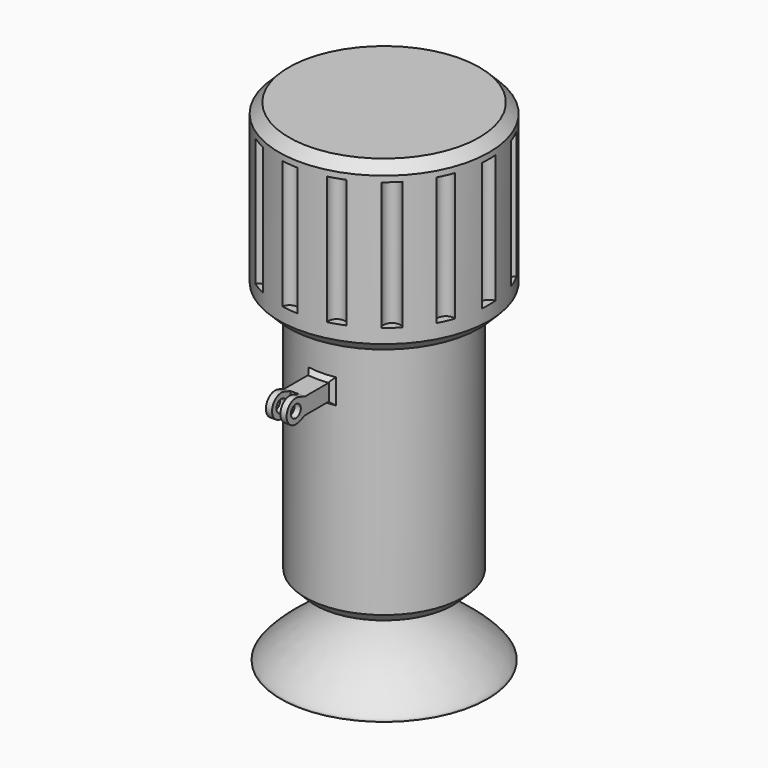
from build123d import *

# Parameters (mm, degrees)
F0_R           = 127
F1_DEPTH       = 254
F2_R           = 127
F2_R_2         = 95.25
F3_DEPTH       = 304.8
F6_R           = 8
F7_DEPTH       = 110
F10_SIZE       = 12
F13_DEPTH      = 155
F15_DEPTH      = 20
F17_DEPTH      = 25
F18_T1_DEPTH   = 20
F18_T6_ANGLE   = 30.5513976385
F18_T12_ANGLE  = 30.5513976385
F18_T18_ANGLE  = 30.5513976385
F18_T24_ANGLE  = 30.5513976385
F18_T31_ANGLE  = 30.5513976385
F18_T35_DEPTH  = 31.0991303205
F18_T42_DEPTH  = 31.0991303205
F18_T46_ANGLE  = 30.5513976385
F18_T53_DEPTH  = 31.0991303205
F18_T57_ANGLE  = 30.5513976385
F18_T64_DEPTH  = 31.0991303205
F18_T68_ANGLE  = 30.5513976385
F18_T75_ANGLE  = 30.5513976385
F18_T79_DEPTH  = 31.0991303205
F18_T86_DEPTH  = 31.0991303205
F18_T90_ANGLE  = 30.5513976385
F18_T97_DEPTH  = 31.0991303205
F18_T101_ANGLE = 30.5513976385
F18_T108_DEPTH = 31.0991303205
F18_T112_ANGLE = 30.5513976385
F19_R          = 7.5
F20_DEPTH      = 25
F23_DEPTH      = 5


# Not quite as in the source:
# - a fillet or chamfer that OpenCascade refuses, or shapes differently, is made with other operations: its cross-section is extruded or revolved along the edge and cut away or added


with BuildPart() as f1:
    # F0 (on Top) → F1 (new body, symmetric)
    with BuildSketch(Plane.XY):
        Circle(F0_R)
    extrude(amount=F1_DEPTH, both=True)

    # F2 (on face) → F3 (cut)
    with BuildSketch(Plane(origin=(0, 0, -254), x_dir=(1, 0, 0), z_dir=(0, 0, -1))):
        Circle(F2_R)
        Circle(F2_R_2, mode=Mode.SUBTRACT)
    extrude(amount=-F3_DEPTH, mode=Mode.SUBTRACT)

    # F4 (on Front) → F5 (revolve)
    with BuildSketch(Plane.XZ):
        with BuildLine():
            Line((8, -272), (8, -254))
            Line((8, -254), (0, -254))
            Line((0, -254), (0, -279))
            add(Edge.make_bspline(
                [(0, -279), (11.9869346113, -279.619316661), (39.0233605765, -281.0161799623), (88.3278716399, -305.4905672545), (123.6075273001, -336.3998966271), (124.6345471897, -339.4650682793), (124.962721218, -340.0125261312), (125.0836998224, -340.2143418789)],
                knots=[0, 0, 0, 0, 0.2695655664, 0.6080027726, 0.8979150102, 0.9623672243, 1, 1, 1, 1], degree=3))
            add(Edge.make_bspline(
                [(8, -272), (33.2367625522, -279.0458738752), (79.549956163, -291.9760950264), (125.9374548971, -335.9181149736), (125.2107880958, -339.5748141321), (125.0836998224, -340.2143418789)],
                knots=[0, 0, 0, 0, 0.4969763521, 0.9120251445, 1, 1, 1, 1], degree=3))
        make_face()
    revolve(axis=Axis((0, 0, -266.5), (0, 0, -1)))

    # F6 (on face) → F7 (join)
    with BuildSketch(Plane(origin=(0, 0, -254), x_dir=(1, 0, 0), z_dir=(0, 0, -1))):
        Circle(F6_R)
    extrude(amount=F7_DEPTH)

    # F10
    f10_edges = [f1.edges().sort_by_distance(p)[0] for p in [
        (-95.25, 0, -254),
        (-127, 0, 254),
        (-127, 0, 50.8),
    ]]
    chamfer(f10_edges, length=F10_SIZE)

    # F12 (on offset) → F13 (cut)
    with BuildSketch(Plane.XY.offset(80)):
        with BuildLine():
            ThreePointArc((111.5963965616, 60.6237929733), (106.8848185442, 47.5881872399), (119.7248225476, 42.3670492946))
            ThreePointArc((119.7248225476, 42.3670492946), (116.0202731206, 51.6555536706), (111.5963965616, 60.6237929733))
        make_face()
        with BuildLine():
            ThreePointArc((126.6062992126, -9.992246979), (127, 0), (126.6062992126, 9.992246979))
            ThreePointArc((126.6062992126, 9.992246979), (117, 0), (126.6062992126, -9.992246979))
        make_face()
        with BuildLine():
            ThreePointArc((92.1418363983, 87.4006978527), (84.9795870076, 94.3793928356), (77.2904631236, 100.7729344127))
            ThreePointArc((77.2904631236, 100.7729344127), (78.288280944, 86.9479445809), (92.1418363983, 87.4006978527))
        make_face()
        with BuildLine():
            ThreePointArc((48.6266896535, 117.3219717416), (39.2451582856, 120.7841775695), (29.6203064498, 123.4975199987))
            ThreePointArc((29.6203064498, 123.4975199987), (36.1549883419, 111.2736124065), (48.6266896535, 117.3219717416))
        make_face()
        with BuildLine():
            ThreePointArc((-3.2964534921, 126.9572108798), (-13.275114835, 126.3042807118), (-23.1714703013, 124.8682624372))
            ThreePointArc((-23.1714703013, 124.8682624372), (-12.2298302023, 116.3590617581), (-3.2964534921, 126.9572108798))
        make_face()
        with BuildLine():
            ThreePointArc((-54.6496098816, 114.6403948868), (-63.5, 109.9852262806), (-71.956689331, 104.6481479077))
            ThreePointArc((-71.956689331, 104.6481479077), (-58.5, 101.3249722428), (-54.6496098816, 114.6403948868))
        make_face()
        with BuildLine():
            ThreePointArc((-96.5533522464, 82.5012131425), (-102.7451582856, 74.6487270411), (-108.2999430695, 66.3334179065))
            ThreePointArc((-108.2999430695, 66.3334179065), (-94.6549883419, 68.7708745182), (-96.5533522464, 82.5012131425))
        make_face()
        with BuildLine():
            ThreePointArc((-121.7621428481, 36.096822146), (-124.2247452932, 26.4047847339), (-125.9171527771, 16.549037329))
            ThreePointArc((-125.9171527771, 16.549037329), (-114.4432692859, 24.3256678257), (-121.7621428481, 36.096822146))
        make_face()
        with BuildLine():
            ThreePointArc((-125.9171527771, -16.549037329), (-124.2247452932, -26.4047847339), (-121.7621428481, -36.096822146))
            ThreePointArc((-121.7621428481, -36.096822146), (-114.4432692859, -24.3256678257), (-125.9171527771, -16.549037329))
        make_face()
        with BuildLine():
            ThreePointArc((-108.2999430695, -66.3334179065), (-102.7451582856, -74.6487270411), (-96.5533522464, -82.5012131425))
            ThreePointArc((-96.5533522464, -82.5012131425), (-94.6549883419, -68.7708745182), (-108.2999430695, -66.3334179065))
        make_face()
        with BuildLine():
            ThreePointArc((-71.956689331, -104.6481479077), (-63.5, -109.9852262806), (-54.6496098816, -114.6403948868))
            ThreePointArc((-54.6496098816, -114.6403948868), (-58.5, -101.3249722428), (-71.956689331, -104.6481479077))
        make_face()
        with BuildLine():
            ThreePointArc((-23.1714703013, -124.8682624372), (-13.275114835, -126.3042807118), (-3.2964534921, -126.9572108798))
            ThreePointArc((-3.2964534921, -126.9572108798), (-12.2298302023, -116.3590617581), (-23.1714703013, -124.8682624372))
        make_face()
        with BuildLine():
            ThreePointArc((29.6203064498, -123.4975199987), (39.2451582856, -120.7841775695), (48.6266896535, -117.3219717416))
            ThreePointArc((48.6266896535, -117.3219717416), (36.1549883419, -111.2736124065), (29.6203064498, -123.4975199987))
        make_face()
        with BuildLine():
            ThreePointArc((77.2904631236, -100.7729344127), (84.9795870076, -94.3793928356), (92.1418363983, -87.4006978527))
            ThreePointArc((92.1418363983, -87.4006978527), (78.288280944, -86.9479445809), (77.2904631236, -100.7729344127))
        make_face()
        with BuildLine():
            ThreePointArc((111.5963965616, -60.6237929733), (116.0202731206, -51.6555536706), (119.7248225476, -42.3670492946))
            ThreePointArc((119.7248225476, -42.3670492946), (106.8848185442, -47.5881872399), (111.5963965616, -60.6237929733))
        make_face()
    extrude(amount=F13_DEPTH, mode=Mode.SUBTRACT)

    # F14 (on Top) → F15 (join)
    with BuildSketch(Plane.XY):
        with BuildLine():
            ThreePointArc((-12.5, 94.1740410092), (0, 95), (12.5, 94.1740410092))
            Line((12.5, 94.1740410092), (12.5, 135))
            Line((12.5, 135), (-12.5, 135))
            Line((-12.5, 135), (-12.5, 94.1740410092))
        make_face()
        with BuildLine():
            ThreePointArc((12.5, -94.1740410092), (0, -95), (-12.5, -94.1740410092))
            Line((-12.5, -94.1740410092), (-12.5, -135))
            Line((-12.5, -135), (12.5, -135))
            Line((12.5, -135), (12.5, -94.1740410092))
        make_face()
    extrude(amount=-F15_DEPTH)

    # F16 (on face) → F17 (join, through all)
    with BuildSketch(Plane(origin=(-12.5, 0, 0), x_dir=(0, -1, 0), z_dir=(-1, 0, 0))):
        with BuildLine():
            Line((135, -20), (144.4594594595, -23.2432432432))
            ThreePointArc((144.4594594595, -23.2432432432), (163, -10), (144.4594594595, 3.2432432432))
            Line((144.4594594595, 3.2432432432), (135, 0))
            Line((135, 0), (135, -20))
        make_face()
        with BuildLine():
            Line((-144.4594594595, -23.2432432432), (-135, -20))
            Line((-135, -20), (-135, 0))
            Line((-135, 0), (-144.4594594595, 3.2432432432))
            ThreePointArc((-144.4594594595, 3.2432432432), (-163, -10), (-144.4594594595, -23.2432432432))
        make_face()
    extrude(amount=-F17_DEPTH)

    # F18: chamfer of 5 on 8 edges, made by hand

    # F18_s2 → F18_t1 (join)
    with BuildSketch(Plane.XY.offset(-20)):
        with BuildLine():
            Line((-16.6271820449, -93.7875221831), (-12.5, -98.710751694))
            Line((-12.5, -98.710751694), (-12.5, -94.4262278183))
            ThreePointArc((-12.5, -94.4262278183), (-14.6414795672, -94.1179556519), (-16.6271820449, -93.7875221831))
        make_face()
        with BuildLine():
            Line((16.6271820449, -93.7875221831), (12.5, -98.710751694))
            Line((12.5, -98.710751694), (12.5, -94.4262278183))
            ThreePointArc((12.5, -94.4262278183), (14.6414795672, -94.1179556519), (16.6271820449, -93.7875221831))
        make_face()
        with BuildLine():
            Line((-16.6271820449, 93.7875221831), (-12.5, 98.710751694))
            Line((-12.5, 98.710751694), (-12.5, 94.4262278183))
            ThreePointArc((-12.5, 94.4262278183), (-14.6414795672, 94.1179556519), (-16.6271820449, 93.7875221831))
        make_face()
        with BuildLine():
            Line((16.6271820449, 93.7875221831), (12.5, 98.710751694))
            Line((12.5, 98.710751694), (12.5, 94.4262278183))
            ThreePointArc((12.5, 94.4262278183), (14.6414795672, 94.1179556519), (16.6271820449, 93.7875221831))
        make_face()
    extrude(amount=F18_T1_DEPTH)


with BuildPart() as f9:
    # F8 (on Front) → F9 (revolve)
    with BuildSketch(Plane.XZ):
        with BuildLine():
            Line((0, -389), (0, -364))
            ThreePointArc((0, -364), (-12.5, -376.5), (0, -389))
        make_face()
    revolve(axis=Axis((0, 0, -376.5), (0, 0, -1)))


with BuildPart() as f18_tool4:
    # F18_s5 → F18_t6 (revolve)
    with BuildSketch(Plane(origin=(0, 0, 0), x_dir=(0, 0, 1), z_dir=(0.9646692497, 0.2634639231, 0))):
        Polygon((-25, 95.25), (-20, 100.25), (-20, 95.25), align=None)
    revolve(axis=Axis((0, 0, -20), (0, 0, -1)), revolution_arc=F18_T6_ANGLE)

    split(bisect_by=Plane.YZ.offset(-12.5), keep=Keep.TOP)

    split(bisect_by=Plane.YZ.offset(12.5), keep=Keep.BOTTOM)


with BuildPart() as f1_1:
    add(f1.part)

    # F18_t3: union F18_tool4
    add(f18_tool4.part)


with BuildPart() as f18_tool10:
    # F18_s11 → F18_t12 (revolve)
    with BuildSketch(Plane(origin=(0, 0, 0), x_dir=(0, 0, 1), z_dir=(0.9646692497, 0.2634639231, 0))):
        Polygon((5, 95.25), (0, 100.25), (0, 95.25), align=None)
    revolve(axis=Axis((0, 0, 0), (0, 0, -1)), revolution_arc=F18_T12_ANGLE)

    split(bisect_by=Plane.YZ.offset(-12.5), keep=Keep.TOP)

    split(bisect_by=Plane.YZ.offset(12.5), keep=Keep.BOTTOM)


with BuildPart() as f1_2:
    add(f1_1.part)

    # F18_t9: union F18_tool10
    add(f18_tool10.part)


with BuildPart() as f18_tool16:
    # F18_s17 → F18_t18 (revolve)
    with BuildSketch(Plane(origin=(0, 0, 0), x_dir=(0, 0, 1), z_dir=(-0.9646692497, -0.2634639231, 0))):
        Polygon((-25, 95.25), (-20, 100.25), (-20, 95.25), align=None)
    revolve(axis=Axis((0, 0, -20), (0, 0, -1)), revolution_arc=F18_T18_ANGLE)

    split(bisect_by=Plane.YZ.offset(12.5), keep=Keep.BOTTOM)

    split(bisect_by=Plane.YZ.offset(-12.5), keep=Keep.TOP)


with BuildPart() as f1_3:
    add(f1_2.part)

    # F18_t15: union F18_tool16
    add(f18_tool16.part)


with BuildPart() as f18_tool22:
    # F18_s23 → F18_t24 (revolve)
    with BuildSketch(Plane(origin=(0, 0, 0), x_dir=(0, 0, 1), z_dir=(-0.9646692497, -0.2634639231, 0))):
        Polygon((5, 95.25), (0, 100.25), (0, 95.25), align=None)
    revolve(axis=Axis((0, 0, 0), (0, 0, -1)), revolution_arc=F18_T24_ANGLE)

    split(bisect_by=Plane.YZ.offset(12.5), keep=Keep.BOTTOM)

    split(bisect_by=Plane.YZ.offset(-12.5), keep=Keep.TOP)


with BuildPart() as f1_4:
    add(f1_3.part)

    # F18_t21: union F18_tool22
    add(f18_tool22.part)


with BuildPart() as f18_tool29:
    # F18_s30 → F18_t31 (revolve)
    with BuildSketch(Plane(origin=(0, 0, 0), x_dir=(0, 0, 1), z_dir=(0.9646692497, 0.2634639231, 0))):
        Polygon((-25, 95.25), (-20, 100.25), (-20, 95.25), align=None)
    revolve(axis=Axis((0, 0, -20), (0, 0, -1)), revolution_arc=F18_T31_ANGLE)

    split(bisect_by=Plane.YZ.offset(12.5), keep=Keep.TOP)


with BuildPart() as f18_tool33:
    # F18_s34 → F18_t35 (new body)
    with BuildSketch(Plane.XY):
        with BuildLine():
            Line((16.6271820449, -93.7875221831), (12.5, -98.710751694))
            Line((12.5, -98.710751694), (12.5, -94.4262278183))
            ThreePointArc((12.5, -94.4262278183), (14.6414795672, -94.1179556519), (16.6271820449, -93.7875221831))
        make_face()
    extrude(amount=-F18_T35_DEPTH)

    split(bisect_by=Plane.XY.offset(-20), keep=Keep.BOTTOM)


with BuildPart() as f18_tool29_1:
    add(f18_tool29.part)

    # F18_t37: intersect F18_tool33
    add(f18_tool33.part, mode=Mode.INTERSECT)


with BuildPart() as f1_5:
    add(f1_4.part)

    # F18_t27: union F18_tool29
    add(f18_tool29_1.part)


with BuildPart() as f18_tool40:
    # F18_s41 → F18_t42 (new body)
    with BuildSketch(Plane.XY):
        with BuildLine():
            Line((-16.6271820449, -93.7875221831), (-12.5, -98.710751694))
            Line((-12.5, -98.710751694), (-12.5, -94.4262278183))
            ThreePointArc((-12.5, -94.4262278183), (-14.6414795672, -94.1179556519), (-16.6271820449, -93.7875221831))
        make_face()
    extrude(amount=-F18_T42_DEPTH)

    split(bisect_by=Plane.XY.offset(-20), keep=Keep.BOTTOM)


with BuildPart() as f18_tool44:
    # F18_s45 → F18_t46 (revolve)
    with BuildSketch(Plane(origin=(0, 0, 0), x_dir=(0, 0, 1), z_dir=(0.9646692497, 0.2634639231, 0))):
        Polygon((-25, 95.25), (-20, 100.25), (-20, 95.25), align=None)
    revolve(axis=Axis((0, 0, -20), (0, 0, -1)), revolution_arc=F18_T46_ANGLE)

    split(bisect_by=Plane.YZ.offset(-12.5), keep=Keep.BOTTOM)


with BuildPart() as f18_tool40_1:
    add(f18_tool40.part)

    # F18_t48: intersect F18_tool44
    add(f18_tool44.part, mode=Mode.INTERSECT)


with BuildPart() as f1_6:
    add(f1_5.part)

    # F18_t38: union F18_tool40
    add(f18_tool40_1.part)


with BuildPart() as f18_tool51:
    # F18_s52 → F18_t53 (new body)
    with BuildSketch(Plane.XY.offset(11.0991303205)):
        with BuildLine():
            Line((-16.6271820449, -93.7875221831), (-12.5, -98.710751694))
            Line((-12.5, -98.710751694), (-12.5, -94.4262278183))
            ThreePointArc((-12.5, -94.4262278183), (-14.6414795672, -94.1179556519), (-16.6271820449, -93.7875221831))
        make_face()
    extrude(amount=-F18_T53_DEPTH)

    split(bisect_by=Plane.XY, keep=Keep.TOP)


with BuildPart() as f18_tool55:
    # F18_s56 → F18_t57 (revolve)
    with BuildSketch(Plane(origin=(0, 0, 0), x_dir=(0, 0, 1), z_dir=(0.9646692497, 0.2634639231, 0))):
        Polygon((5, 95.25), (0, 100.25), (0, 95.25), align=None)
    revolve(axis=Axis((0, 0, 0), (0, 0, -1)), revolution_arc=F18_T57_ANGLE)

    split(bisect_by=Plane.YZ.offset(-12.5), keep=Keep.BOTTOM)


with BuildPart() as f18_tool51_1:
    add(f18_tool51.part)

    # F18_t59: intersect F18_tool55
    add(f18_tool55.part, mode=Mode.INTERSECT)


with BuildPart() as f1_7:
    add(f1_6.part)

    # F18_t49: union F18_tool51
    add(f18_tool51_1.part)


with BuildPart() as f18_tool62:
    # F18_s63 → F18_t64 (new body)
    with BuildSketch(Plane.XY.offset(11.0991303205)):
        with BuildLine():
            Line((16.6271820449, -93.7875221831), (12.5, -98.710751694))
            Line((12.5, -98.710751694), (12.5, -94.4262278183))
            ThreePointArc((12.5, -94.4262278183), (14.6414795672, -94.1179556519), (16.6271820449, -93.7875221831))
        make_face()
    extrude(amount=-F18_T64_DEPTH)

    split(bisect_by=Plane.XY, keep=Keep.TOP)


with BuildPart() as f18_tool66:
    # F18_s67 → F18_t68 (revolve)
    with BuildSketch(Plane(origin=(0, 0, 0), x_dir=(0, 0, 1), z_dir=(0.9646692497, 0.2634639231, 0))):
        Polygon((5, 95.25), (0, 100.25), (0, 95.25), align=None)
    revolve(axis=Axis((0, 0, 0), (0, 0, -1)), revolution_arc=F18_T68_ANGLE)

    split(bisect_by=Plane.YZ.offset(12.5), keep=Keep.TOP)


with BuildPart() as f18_tool62_1:
    add(f18_tool62.part)

    # F18_t70: intersect F18_tool66
    add(f18_tool66.part, mode=Mode.INTERSECT)


with BuildPart() as f1_8:
    add(f1_7.part)

    # F18_t60: union F18_tool62
    add(f18_tool62_1.part)


with BuildPart() as f18_tool73:
    # F18_s74 → F18_t75 (revolve)
    with BuildSketch(Plane(origin=(0, 0, 0), x_dir=(0, 0, 1), z_dir=(-0.9646692497, -0.2634639231, 0))):
        Polygon((-25, 95.25), (-20, 100.25), (-20, 95.25), align=None)
    revolve(axis=Axis((0, 0, -20), (0, 0, -1)), revolution_arc=F18_T75_ANGLE)

    split(bisect_by=Plane.YZ.offset(-12.5), keep=Keep.BOTTOM)


with BuildPart() as f18_tool77:
    # F18_s78 → F18_t79 (new body)
    with BuildSketch(Plane.XY):
        with BuildLine():
            Line((-16.6271820449, 93.7875221831), (-12.5, 98.710751694))
            Line((-12.5, 98.710751694), (-12.5, 94.4262278183))
            ThreePointArc((-12.5, 94.4262278183), (-14.6414795672, 94.1179556519), (-16.6271820449, 93.7875221831))
        make_face()
    extrude(amount=-F18_T79_DEPTH)

    split(bisect_by=Plane.XY.offset(-20), keep=Keep.BOTTOM)


with BuildPart() as f18_tool73_1:
    add(f18_tool73.part)

    # F18_t81: intersect F18_tool77
    add(f18_tool77.part, mode=Mode.INTERSECT)


with BuildPart() as f1_9:
    add(f1_8.part)

    # F18_t71: union F18_tool73
    add(f18_tool73_1.part)


with BuildPart() as f18_tool84:
    # F18_s85 → F18_t86 (new body)
    with BuildSketch(Plane.XY):
        with BuildLine():
            Line((16.6271820449, 93.7875221831), (12.5, 98.710751694))
            Line((12.5, 98.710751694), (12.5, 94.4262278183))
            ThreePointArc((12.5, 94.4262278183), (14.6414795672, 94.1179556519), (16.6271820449, 93.7875221831))
        make_face()
    extrude(amount=-F18_T86_DEPTH)

    split(bisect_by=Plane.XY.offset(-20), keep=Keep.BOTTOM)


with BuildPart() as f18_tool88:
    # F18_s89 → F18_t90 (revolve)
    with BuildSketch(Plane(origin=(0, 0, 0), x_dir=(0, 0, 1), z_dir=(-0.9646692497, -0.2634639231, 0))):
        Polygon((-25, 95.25), (-20, 100.25), (-20, 95.25), align=None)
    revolve(axis=Axis((0, 0, -20), (0, 0, -1)), revolution_arc=F18_T90_ANGLE)

    split(bisect_by=Plane.YZ.offset(12.5), keep=Keep.TOP)


with BuildPart() as f18_tool84_1:
    add(f18_tool84.part)

    # F18_t92: intersect F18_tool88
    add(f18_tool88.part, mode=Mode.INTERSECT)


with BuildPart() as f1_10:
    add(f1_9.part)

    # F18_t82: union F18_tool84
    add(f18_tool84_1.part)


with BuildPart() as f18_tool95:
    # F18_s96 → F18_t97 (new body)
    with BuildSketch(Plane.XY.offset(11.0991303205)):
        with BuildLine():
            Line((-16.6271820449, 93.7875221831), (-12.5, 98.710751694))
            Line((-12.5, 98.710751694), (-12.5, 94.4262278183))
            ThreePointArc((-12.5, 94.4262278183), (-14.6414795672, 94.1179556519), (-16.6271820449, 93.7875221831))
        make_face()
    extrude(amount=-F18_T97_DEPTH)

    split(bisect_by=Plane.XY, keep=Keep.TOP)


with BuildPart() as f18_tool99:
    # F18_s100 → F18_t101 (revolve)
    with BuildSketch(Plane(origin=(0, 0, 0), x_dir=(0, 0, 1), z_dir=(-0.9646692497, -0.2634639231, 0))):
        Polygon((5, 95.25), (0, 100.25), (0, 95.25), align=None)
    revolve(axis=Axis((0, 0, 0), (0, 0, -1)), revolution_arc=F18_T101_ANGLE)

    split(bisect_by=Plane.YZ.offset(-12.5), keep=Keep.BOTTOM)


with BuildPart() as f18_tool95_1:
    add(f18_tool95.part)

    # F18_t103: intersect F18_tool99
    add(f18_tool99.part, mode=Mode.INTERSECT)


with BuildPart() as f1_11:
    add(f1_10.part)

    # F18_t93: union F18_tool95
    add(f18_tool95_1.part)


with BuildPart() as f18_tool106:
    # F18_s107 → F18_t108 (new body)
    with BuildSketch(Plane.XY.offset(11.0991303205)):
        with BuildLine():
            Line((16.6271820449, 93.7875221831), (12.5, 98.710751694))
            Line((12.5, 98.710751694), (12.5, 94.4262278183))
            ThreePointArc((12.5, 94.4262278183), (14.6414795672, 94.1179556519), (16.6271820449, 93.7875221831))
        make_face()
    extrude(amount=-F18_T108_DEPTH)

    split(bisect_by=Plane.XY, keep=Keep.TOP)


with BuildPart() as f18_tool110:
    # F18_s111 → F18_t112 (revolve)
    with BuildSketch(Plane(origin=(0, 0, 0), x_dir=(0, 0, 1), z_dir=(-0.9646692497, -0.2634639231, 0))):
        Polygon((5, 95.25), (0, 100.25), (0, 95.25), align=None)
    revolve(axis=Axis((0, 0, 0), (0, 0, -1)), revolution_arc=F18_T112_ANGLE)

    split(bisect_by=Plane.YZ.offset(12.5), keep=Keep.TOP)


with BuildPart() as f18_tool106_1:
    add(f18_tool106.part)

    # F18_t114: intersect F18_tool110
    add(f18_tool110.part, mode=Mode.INTERSECT)


with BuildPart() as f1_12:
    add(f1_11.part)

    # F18_t104: union F18_tool106
    add(f18_tool106_1.part)

    # F19 (on face) → F20 (cut)
    with BuildSketch(Plane.YZ.offset(12.5)):
        with Locations((149, -10)):
            Circle(F19_R)
        with Locations((-149, -10)):
            Circle(F19_R)
    extrude(amount=-F20_DEPTH, mode=Mode.SUBTRACT)

    # F22 (on mid) → F23 (cut, symmetric)
    with BuildSketch(Plane.YZ):
        with BuildLine():
            ThreePointArc((144.4594594595, -23.2432432432), (163, -10), (144.4594594595, 3.2432432432))
            Line((144.4594594595, 3.2432432432), (135, 0))
            Line((135, 0), (135, -20))
            Line((135, -20), (144.4594594595, -23.2432432432))
        make_face()
        with BuildLine():
            Line((-144.4594594595, -23.2432432432), (-135, -20))
            Line((-135, -20), (-135, 0))
            Line((-135, 0), (-144.4594594595, 3.2432432432))
            ThreePointArc((-144.4594594595, 3.2432432432), (-163, -10), (-144.4594594595, -23.2432432432))
        make_face()
    extrude(amount=F23_DEPTH, both=True, mode=Mode.SUBTRACT)


solid = Compound([f9.part, f1_12.part])
